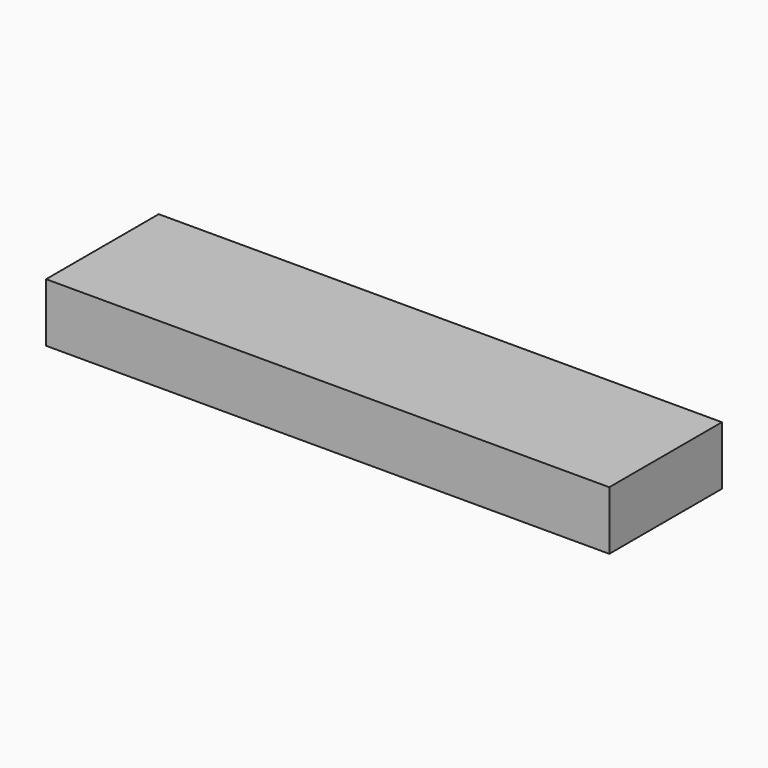
from build123d import *

# Parameters (mm, degrees)
F0_W     = 152.4
F0_H     = 38.1
F1_DEPTH = 15.875


# Not quite as in the source:
# - a length typed as a fraction of an inch, garbled in the dataset ("3 / 203.2 mm" for 3/8 in), is restored


with BuildPart() as f1:
    # F0 (on Top) → F1 (new body)
    with BuildSketch(Plane.XY):
        Rectangle(F0_W, F0_H)
    extrude(amount=F1_DEPTH)


solid = f1.part
